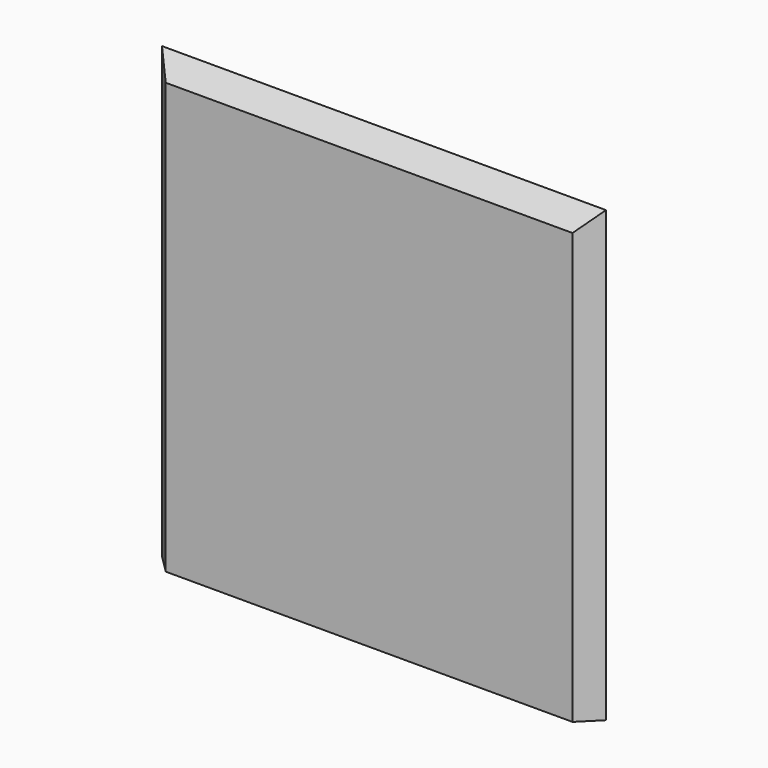
from build123d import *

# Parameters (mm, degrees)
F0_W        = 195
F0_H        = 195
F1_DEPTH    = 4.0000047
F2_T1_DEPTH = 247.2565983155
F3_T1_DEPTH = 247.2565983155
F4_T1_DEPTH = 226.9365983155


# Not quite as in the source:
# - a fillet or chamfer that OpenCascade refuses, or shapes differently, is made with other operations: its cross-section is extruded or revolved along the edge and cut away or added


with BuildPart() as f1:
    # F0 (on Front) → F1 (new body, symmetric)
    with BuildSketch(Plane.XZ):
        Rectangle(F0_W, F0_H)
    extrude(amount=F1_DEPTH, both=True)

    # F2: chamfer of 10.16 on 1 edges, made by hand

    # F2_s2 → F2_t1 (cut)
    with BuildSketch(Plane.XY.offset(-123.6282991577)):
        Polygon((97.5, 6.1599953), (87.34, -4.0000047), (97.5, -4.0000047), align=None)
    extrude(amount=F2_T1_DEPTH, mode=Mode.SUBTRACT)

    # F3: chamfer of 10.16 on 1 edges, made by hand

    # F3_s2 → F3_t1 (cut)
    with BuildSketch(Plane.XY.offset(-123.6282991577)):
        Polygon((-97.5, 6.1599953), (-87.34, -4.0000047), (-97.5, -4.0000047), align=None)
    extrude(amount=F3_T1_DEPTH, mode=Mode.SUBTRACT)

    # F4: chamfer of 10.16 on 1 edges, made by hand

    # F4_s2 → F4_t1 (cut)
    with BuildSketch(Plane.YZ.offset(-113.4682991577)):
        Polygon((6.1599953, 97.5), (-4.0000047, 87.34), (-4.0000047, 97.5), align=None)
    extrude(amount=F4_T1_DEPTH, mode=Mode.SUBTRACT)


solid = f1.part
